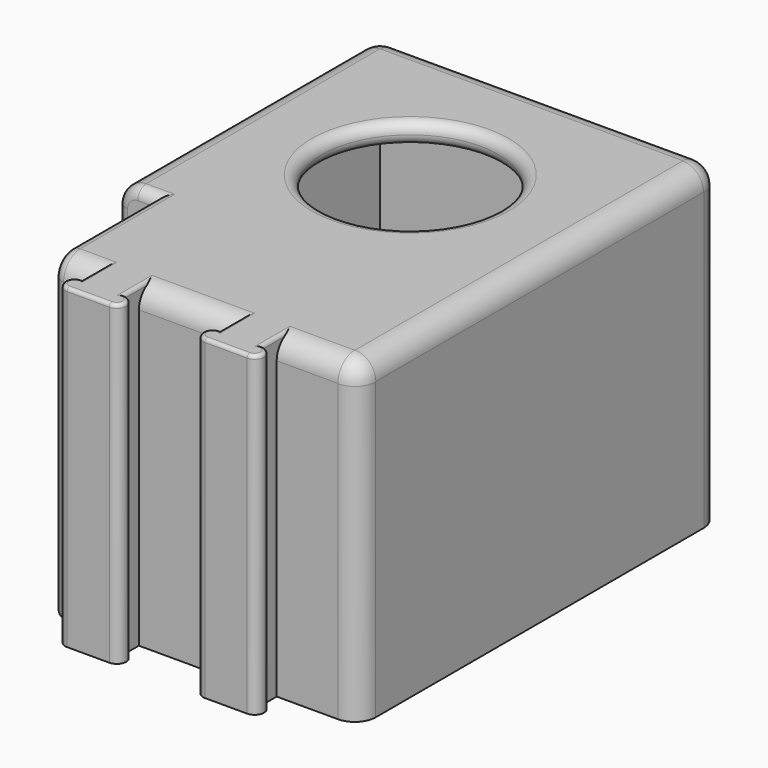
from build123d import *

# Parameters (mm, degrees)
F0_W           = 49
F0_H           = 49
F0_W_2         = 43
F0_H_2         = 43
F1_DEPTH       = 42
F2_DEPTH       = 3
F3_R           = 12.5
F4_DEPTH       = 3.001
F5_W           = 17
F5_H           = 13
F6_DEPTH       = 24.501
F8_DEPTH       = 42
F7_W           = 43
F7_H           = 12.25
F9_DEPTH       = 3
F11_DEPTH      = 3
F11_DEPTH_BACK = 42
F13_W          = 18.25
F13_H          = 45
F14_DEPTH      = 5.5
F15_T4_DEPTH   = 49.5024142802
F15_T9_DEPTH   = 48.0024142802
F15_T14_DEPTH  = 48.0024142802
F15_T19_DEPTH  = 49.5024142802
F15_T21_DEPTH  = 49.5014485948
F15_T23_DEPTH  = 50.5014485948
F15_T25_DEPTH  = 58.2480686292
F15_T27_DEPTH  = 42.9980686292
F15_T29_DEPTH  = 8.6990343146
F15_T31_DEPTH  = 13.7024142802
F15_T33_DEPTH  = 13.6
F15_S37_W      = 3.3015022539
F15_S37_H      = 3.3015022539
F15_T38_DEPTH  = 3.301502254
F15_S43_W      = 3.3015022539
F15_S43_H      = 3.3015022539
F15_T44_DEPTH  = 3.301502254
F15_S49_W      = 3.3015022539
F15_S49_H      = 3.3015022539
F15_T50_DEPTH  = 3.301502254
F15_T56_DEPTH  = 16.2014485948
F15_T61_DEPTH  = 21.2048285604
F15_T66_DEPTH  = 28.6048285604
F15_T71_DEPTH  = 28.6048285604
F16_R          = 1.49999
F17_R          = 1.5
F18_R          = 0.5


# Not quite as in the source:
# - a fillet or chamfer that OpenCascade refuses, or shapes differently, is made with other operations: its cross-section is extruded or revolved along the edge and cut away or added
# - a fillet or chamfer is up to 0.001 mm smaller than in the source, because OpenCascade refuses the exact size
# - a pattern or mirror of a feature is missing from the dataset's text; its kind, count and spacing are read off the source's solid


with BuildPart() as f1:
    # F0 (on Top) → F1 (new body)
    with BuildSketch(Plane.XY):
        Rectangle(F0_W, F0_H)
        Rectangle(F0_W_2, F0_H_2, mode=Mode.SUBTRACT)
    extrude(amount=-F1_DEPTH)

    # F0 (on Top) → F2 (join)
    with BuildSketch(Plane.XY):
        Rectangle(F0_W, F0_H)
        Rectangle(F0_W_2, F0_H_2, mode=Mode.SUBTRACT)
        Rectangle(F0_W_2, F0_H_2)
    extrude(amount=F2_DEPTH)

    # F3 (on Top) → F4 (cut, through all)
    with BuildSketch(Plane.XY):
        Circle(F3_R)
    extrude(amount=F4_DEPTH, mode=Mode.SUBTRACT)

    # F5 (on Front) → F6 (cut, through all)
    with BuildSketch(Plane.XZ):
        with Locations((0, -35.5)):
            Rectangle(F5_W, F5_H)
    extrude(amount=-F6_DEPTH, mode=Mode.SUBTRACT)

    # F7 (on Top) → F8 (join, through all)
    with BuildSketch(Plane.XY):
        Polygon((-21.5, -24.5), (-24.5, -24.5), (-24.5, -39.75), (24.5, -39.75), (24.5, -24.5), (21.5, -24.5), (21.5, -36.75), (-21.5, -36.75), align=None)
    extrude(amount=-F8_DEPTH)

    # F7 (on Top) → F9 (join, through all)
    with BuildSketch(Plane.XY):
        with Locations((0, -30.625)):
            Rectangle(F7_W, F7_H)
        Polygon((-21.5, -24.5), (-24.5, -24.5), (-24.5, -39.75), (24.5, -39.75), (24.5, -24.5), (21.5, -24.5), (21.5, -36.75), (-21.5, -36.75), align=None)
    extrude(amount=F9_DEPTH)

    # F10 (on Top) → F11 (join, two sides)
    with BuildSketch(Plane.XY) as f11_sk:
        with BuildLine():
            Line((12.8, -39.75), (6.8, -39.75))
            Line((6.8, -39.75), (6.8, -42.35))
            ThreePointArc((6.8, -42.35), (5.475, -43.675), (6.8, -45))
            Line((6.8, -45), (12.8, -45))
            ThreePointArc((12.8, -45), (14.125, -43.675), (12.8, -42.35))
            Line((12.8, -42.35), (12.8, -39.75))
        make_face()
    f11 = extrude(amount=F11_DEPTH) + extrude(f11_sk.sketch, amount=-F11_DEPTH_BACK)

    # F11_copies: F11 across plane
    add(f11.mirror(Plane(origin=(0, 0, 0), x_dir=(0, 0, -1), z_dir=(-1, 0, 0))))

    # F13 (on offset) → F14 (cut, through all)
    with BuildSketch(Plane.YZ.offset(-19)):
        with Locations((-30.625, -19.5)):
            Rectangle(F13_W, F13_H)
    extrude(amount=-F14_DEPTH, mode=Mode.SUBTRACT)

    # F15: fillet of radius 3 on 13 edges, made by hand


with BuildPart() as f15_tool2:
    # F15_s3 → F15_t4 (new body)
    with BuildSketch(Plane.XY.offset(7.5024142802)):
        with BuildLine():
            ThreePointArc((18.4990343146, -24.4996), (20.6213203436, -25.3786796564), (21.5004, -27.5009656854))
            Line((21.5004, -27.5009656854), (21.8005365685, -27.5009656854))
            ThreePointArc((21.8005365685, -27.5009656854), (21.8001365685, -26.0004828427), (21.8001365685, -24.5))
            Line((21.8001365685, -24.5), (21.5, -24.1998634315))
            ThreePointArc((21.5, -24.1998634315), (19.9995171573, -24.1998634315), (18.4990343146, -24.1994634315))
            Line((18.4990343146, -24.1994634315), (18.4990343146, -24.4996))
        make_face()
    extrude(amount=-F15_T4_DEPTH)

    split(bisect_by=Plane.XY.offset(3), keep=Keep.BOTTOM)


with BuildPart() as f1_1:
    add(f1.part)

    # F15_t1: union F15_tool2
    add(f15_tool2.part)


with BuildPart() as f15_tool7:
    # F15_s8 → F15_t9 (new body)
    with BuildSketch(Plane.YZ.offset(29.0024142802)):
        with BuildLine():
            ThreePointArc((-24.4996, -3.0009656854), (-25.3786796564, -0.8786796564), (-27.5009656854, 0.0004))
            Line((-27.5009656854, 0.0004), (-27.5009656854, 0.3005365685))
            ThreePointArc((-27.5009656854, 0.3005365685), (-26.0004828427, 0.3001365685), (-24.5, 0.3001365685))
            Line((-24.5, 0.3001365685), (-24.1998634315, 0))
            ThreePointArc((-24.1998634315, 0), (-24.1998634315, -1.5004828427), (-24.1994634315, -3.0009656854))
            Line((-24.1994634315, -3.0009656854), (-24.4996, -3.0009656854))
        make_face()
    extrude(amount=-F15_T9_DEPTH)

    split(bisect_by=Plane.YZ.offset(24.5), keep=Keep.BOTTOM)


with BuildPart() as f1_2:
    add(f1_1.part)

    # F15_t6: union F15_tool7
    add(f15_tool7.part)


with BuildPart() as f15_tool12:
    # F15_s13 → F15_t14 (new body)
    with BuildSketch(Plane.YZ.offset(29.0024142802)):
        with BuildLine():
            ThreePointArc((-33.7490343146, 0.0004), (-35.8713203436, -0.8786796564), (-36.7504, -3.0009656854))
            Line((-36.7504, -3.0009656854), (-37.0505365685, -3.0009656854))
            ThreePointArc((-37.0505365685, -3.0009656854), (-37.0501365685, -1.5004828427), (-37.0501365685, 0))
            Line((-37.0501365685, 0), (-36.75, 0.3001365685))
            ThreePointArc((-36.75, 0.3001365685), (-35.2495171573, 0.3001365685), (-33.7490343146, 0.3005365685))
            Line((-33.7490343146, 0.3005365685), (-33.7490343146, 0.0004))
        make_face()
    extrude(amount=-F15_T14_DEPTH)

    split(bisect_by=Plane.YZ.offset(24.5), keep=Keep.BOTTOM)


with BuildPart() as f1_3:
    add(f1_2.part)

    # F15_t11: union F15_tool12
    add(f15_tool12.part)


with BuildPart() as f15_tool17:
    # F15_s18 → F15_t19 (new body)
    with BuildSketch(Plane.XY.offset(7.5024142802)):
        with BuildLine():
            ThreePointArc((21.5004, -33.7490343146), (20.6213203436, -35.8713203436), (18.4990343146, -36.7504))
            Line((18.4990343146, -36.7504), (18.4990343146, -37.0505365685))
            ThreePointArc((18.4990343146, -37.0505365685), (19.9995171573, -37.0501365685), (21.5, -37.0501365685))
            Line((21.5, -37.0501365685), (21.8001365685, -36.75))
            ThreePointArc((21.8001365685, -36.75), (21.8001365685, -35.2495171573), (21.8005365685, -33.7490343146))
            Line((21.8005365685, -33.7490343146), (21.5004, -33.7490343146))
        make_face()
    extrude(amount=-F15_T19_DEPTH)

    split(bisect_by=Plane.XY.offset(3), keep=Keep.BOTTOM)


with BuildPart() as f1_4:
    add(f1_3.part)

    # F15_t16: union F15_tool17
    add(f15_tool17.part)

    # F15_s22 → F15_t21 (cut)
    with BuildSketch(Plane.XY.offset(-49.5024142802)):
        with BuildLine():
            ThreePointArc((21.4990343146, 24.5004), (23.6213203436, 23.6213203436), (24.5004, 21.4990343146))
            Line((24.5004, 21.4990343146), (24.8005365685, 21.4990343146))
            ThreePointArc((24.8005365685, 21.4990343146), (24.8001365685, 22.9995171573), (24.8001365685, 24.5))
            Line((24.8001365685, 24.5), (24.5, 24.8001365685))
            ThreePointArc((24.5, 24.8001365685), (22.9995171573, 24.8001365685), (21.4990343146, 24.8005365685))
            Line((21.4990343146, 24.8005365685), (21.4990343146, 24.5004))
        make_face()
        with BuildLine():
            ThreePointArc((-21.4990343146, 24.5004), (-23.6213203436, 23.6213203436), (-24.5004, 21.4990343146))
            Line((-24.5004, 21.4990343146), (-24.8005365685, 21.4990343146))
            ThreePointArc((-24.8005365685, 21.4990343146), (-24.8001365685, 22.9995171573), (-24.8001365685, 24.5))
            Line((-24.8001365685, 24.5), (-24.5, 24.8001365685))
            ThreePointArc((-24.5, 24.8001365685), (-22.9995171573, 24.8001365685), (-21.4990343146, 24.8005365685))
            Line((-21.4990343146, 24.8005365685), (-21.4990343146, 24.5004))
        make_face()
        with BuildLine():
            ThreePointArc((24.5004, -36.7490343146), (23.6213203436, -38.8713203436), (21.4990343146, -39.7504))
            Line((21.4990343146, -39.7504), (21.4990343146, -40.0505365685))
            ThreePointArc((21.4990343146, -40.0505365685), (22.9995171573, -40.0501365685), (24.5, -40.0501365685))
            Line((24.5, -40.0501365685), (24.8001365685, -39.75))
            ThreePointArc((24.8001365685, -39.75), (24.8001365685, -38.2495171573), (24.8005365685, -36.7490343146))
            Line((24.8005365685, -36.7490343146), (24.5004, -36.7490343146))
        make_face()
    extrude(amount=F15_T21_DEPTH, mode=Mode.SUBTRACT)

    # F15_s24 → F15_t23 (cut)
    with BuildSketch(Plane.XZ.offset(-21.4990343146)):
        with BuildLine():
            ThreePointArc((-21.4990343146, 3.0004), (-23.6213203436, 2.1213203436), (-24.5004, -0.0009656854))
            Line((-24.5004, -0.0009656854), (-24.8005365685, -0.0009656854))
            ThreePointArc((-24.8005365685, -0.0009656854), (-24.8001365685, 1.4995171573), (-24.8001365685, 3))
            Line((-24.8001365685, 3), (-24.5, 3.3001365685))
            ThreePointArc((-24.5, 3.3001365685), (-22.9995171573, 3.3001365685), (-21.4990343146, 3.3005365685))
            Line((-21.4990343146, 3.3005365685), (-21.4990343146, 3.0004))
        make_face()
    extrude(amount=F15_T23_DEPTH, mode=Mode.SUBTRACT)

    # F15_s26 → F15_t25 (cut)
    with BuildSketch(Plane.XZ.offset(-21.4990343146)):
        with BuildLine():
            ThreePointArc((24.5004, -0.0009656854), (23.6213203436, 2.1213203436), (21.4990343146, 3.0004))
            Line((21.4990343146, 3.0004), (21.4990343146, 3.3005365685))
            ThreePointArc((21.4990343146, 3.3005365685), (22.9995171573, 3.3001365685), (24.5, 3.3001365685))
            Line((24.5, 3.3001365685), (24.8001365685, 3))
            ThreePointArc((24.8001365685, 3), (24.8001365685, 1.4995171573), (24.8005365685, -0.0009656854))
            Line((24.8005365685, -0.0009656854), (24.5004, -0.0009656854))
        make_face()
    extrude(amount=F15_T25_DEPTH, mode=Mode.SUBTRACT)

    # F15_s28 → F15_t27 (cut)
    with BuildSketch(Plane.YZ.offset(-21.4990343146)):
        with BuildLine():
            ThreePointArc((24.5004, -0.0009656854), (23.6213203436, 2.1213203436), (21.4990343146, 3.0004))
            Line((21.4990343146, 3.0004), (21.4990343146, 3.3005365685))
            ThreePointArc((21.4990343146, 3.3005365685), (22.9995171573, 3.3001365685), (24.5, 3.3001365685))
            Line((24.5, 3.3001365685), (24.8001365685, 3))
            ThreePointArc((24.8001365685, 3), (24.8001365685, 1.4995171573), (24.8005365685, -0.0009656854))
            Line((24.8005365685, -0.0009656854), (24.5004, -0.0009656854))
        make_face()
    extrude(amount=F15_T27_DEPTH, mode=Mode.SUBTRACT)

    # F15_s30 → F15_t29 (cut)
    with BuildSketch(Plane.YZ.offset(12.8)):
        with BuildLine():
            ThreePointArc((-39.7504, -0.0009656854), (-38.8713203436, 2.1213203436), (-36.7490343146, 3.0004))
            Line((-36.7490343146, 3.0004), (-36.7490343146, 3.3005365685))
            ThreePointArc((-36.7490343146, 3.3005365685), (-38.2495171573, 3.3001365685), (-39.75, 3.3001365685))
            Line((-39.75, 3.3001365685), (-40.0501365685, 3))
            ThreePointArc((-40.0501365685, 3), (-40.0501365685, 1.4995171573), (-40.0505365685, -0.0009656854))
            Line((-40.0505365685, -0.0009656854), (-39.7504, -0.0009656854))
        make_face()
    extrude(amount=F15_T29_DEPTH, mode=Mode.SUBTRACT)

    # F15_s32 → F15_t31 (cut)
    with BuildSketch(Plane.YZ.offset(-26.5024142802)):
        with BuildLine():
            ThreePointArc((-39.7504, -0.0009656854), (-38.8713203436, 2.1213203436), (-36.7490343146, 3.0004))
            Line((-36.7490343146, 3.0004), (-36.7490343146, 3.3005365685))
            ThreePointArc((-36.7490343146, 3.3005365685), (-38.2495171573, 3.3001365685), (-39.75, 3.3001365685))
            Line((-39.75, 3.3001365685), (-40.0501365685, 3))
            ThreePointArc((-40.0501365685, 3), (-40.0501365685, 1.4995171573), (-40.0505365685, -0.0009656854))
            Line((-40.0505365685, -0.0009656854), (-39.7504, -0.0009656854))
        make_face()
    extrude(amount=F15_T31_DEPTH, mode=Mode.SUBTRACT)

    # F15_s34 → F15_t33 (cut)
    with BuildSketch(Plane.YZ.offset(-6.8)):
        with BuildLine():
            ThreePointArc((-39.7504, -0.0009656854), (-38.8713203436, 2.1213203436), (-36.7490343146, 3.0004))
            Line((-36.7490343146, 3.0004), (-36.7490343146, 3.3005365685))
            ThreePointArc((-36.7490343146, 3.3005365685), (-38.2495171573, 3.3001365685), (-39.75, 3.3001365685))
            Line((-39.75, 3.3001365685), (-40.0501365685, 3))
            ThreePointArc((-40.0501365685, 3), (-40.0501365685, 1.4995171573), (-40.0505365685, -0.0009656854))
            Line((-40.0505365685, -0.0009656854), (-39.7504, -0.0009656854))
        make_face()
    extrude(amount=F15_T33_DEPTH, mode=Mode.SUBTRACT)


with BuildPart() as f15_tool36:
    # F15_s37 → F15_t38 (new body)
    with BuildSketch(Plane.XY.offset(-0.0009656854)):
        with Locations((23.1497854416, 23.1497854416)):
            Rectangle(F15_S37_W, F15_S37_H)
    extrude(amount=F15_T38_DEPTH)

    # F15_s39 → F15_t40 (revolve, cut)
    with BuildSketch(Plane(origin=(21.4990343146, 21.4990343146, -0.0009656854), x_dir=(-0.7071067812, -0.7071067812, 0), z_dir=(-0.7071067812, 0.7071067812, 0))):
        with BuildLine():
            ThreePointArc((0, -3.0013656854), (3.0013656854, 0), (0, 3.0013656854))
            Line((0, 3.0013656854), (0, -3.0013656854))
        make_face()
    revolve(axis=Axis((21.4990343146, 21.4990343146, -0.0009656854), (0, 0, 1)), mode=Mode.SUBTRACT)


with BuildPart() as f1_5:
    add(f1_4.part)

    # F15_t35: cut F15_tool36
    add(f15_tool36.part, mode=Mode.SUBTRACT)


with BuildPart() as f15_tool42:
    # F15_s43 → F15_t44 (new body)
    with BuildSketch(Plane.XZ.offset(-21.4990343146)):
        with Locations((-23.1497854416, 1.6497854415)):
            Rectangle(F15_S43_W, F15_S43_H)
    extrude(amount=-F15_T44_DEPTH)

    # F15_s45 → F15_t46 (revolve, cut)
    with BuildSketch(Plane(origin=(-21.4990343146, 21.4990343146, -0.0009656854), x_dir=(0.7071067812, 0, -0.7071067812), z_dir=(0.7071067812, 0, 0.7071067812))):
        with BuildLine():
            ThreePointArc((0, -3.0013656854), (3.0013656854, 0), (0, 3.0013656854))
            Line((0, 3.0013656854), (0, -3.0013656854))
        make_face()
    revolve(axis=Axis((-21.4990343146, 21.4990343146, -0.0009656854), (0, 1, 0)), mode=Mode.SUBTRACT)


with BuildPart() as f1_6:
    add(f1_5.part)

    # F15_t41: cut F15_tool42
    add(f15_tool42.part, mode=Mode.SUBTRACT)


with BuildPart() as f15_tool48:
    # F15_s49 → F15_t50 (new body)
    with BuildSketch(Plane.XY.offset(-0.0009656854)):
        with Locations((23.1497854416, -38.3997854416)):
            Rectangle(F15_S49_W, F15_S49_H)
    extrude(amount=F15_T50_DEPTH)

    # F15_s51 → F15_t52 (revolve, cut)
    with BuildSketch(Plane(origin=(21.4990343146, -36.7490343146, -0.0009656854), x_dir=(-0.7071067812, 0.7071067812, 0), z_dir=(0.7071067812, 0.7071067812, 0))):
        with BuildLine():
            ThreePointArc((0, -3.0013656854), (3.0013656854, 0), (0, 3.0013656854))
            Line((0, 3.0013656854), (0, -3.0013656854))
        make_face()
    revolve(axis=Axis((21.4990343146, -36.7490343146, -0.0009656854), (0, 0, 1)), mode=Mode.SUBTRACT)


with BuildPart() as f1_7:
    add(f1_6.part)

    # F15_t47: cut F15_tool48
    add(f15_tool48.part, mode=Mode.SUBTRACT)


with BuildPart() as f15_tool54:
    # F15_s55 → F15_t56 (new body)
    with BuildSketch(Plane.YZ.offset(5.2975857198)):
        with BuildLine():
            ThreePointArc((-39.7504, -0.0009656854), (-38.8713203436, 2.1213203436), (-36.7490343146, 3.0004))
            Line((-36.7490343146, 3.0004), (-36.7490343146, 3.3005365685))
            ThreePointArc((-36.7490343146, 3.3005365685), (-38.2495171573, 3.3001365685), (-39.75, 3.3001365685))
            Line((-39.75, 3.3001365685), (-40.0501365685, 3))
            ThreePointArc((-40.0501365685, 3), (-40.0501365685, 1.4995171573), (-40.0505365685, -0.0009656854))
            Line((-40.0505365685, -0.0009656854), (-39.7504, -0.0009656854))
        make_face()
    extrude(amount=F15_T56_DEPTH)

    split(bisect_by=Plane.YZ.offset(6.8), keep=Keep.BOTTOM)


with BuildPart() as f1_8:
    add(f1_7.part)

    # F15_t53: cut F15_tool54
    add(f15_tool54.part, mode=Mode.SUBTRACT)


with BuildPart() as f15_tool59:
    # F15_s60 → F15_t61 (new body)
    with BuildSketch(Plane.YZ.offset(-26.5024142802)):
        with BuildLine():
            ThreePointArc((-39.7504, -0.0009656854), (-38.8713203436, 2.1213203436), (-36.7490343146, 3.0004))
            Line((-36.7490343146, 3.0004), (-36.7490343146, 3.3005365685))
            ThreePointArc((-36.7490343146, 3.3005365685), (-38.2495171573, 3.3001365685), (-39.75, 3.3001365685))
            Line((-39.75, 3.3001365685), (-40.0501365685, 3))
            ThreePointArc((-40.0501365685, 3), (-40.0501365685, 1.4995171573), (-40.0505365685, -0.0009656854))
            Line((-40.0505365685, -0.0009656854), (-39.7504, -0.0009656854))
        make_face()
    extrude(amount=F15_T61_DEPTH)

    split(bisect_by=Plane.YZ.offset(-6.8), keep=Keep.TOP)


with BuildPart() as f1_9:
    add(f1_8.part)

    # F15_t58: cut F15_tool59
    add(f15_tool59.part, mode=Mode.SUBTRACT)


with BuildPart() as f15_tool64:
    # F15_s65 → F15_t66 (new body)
    with BuildSketch(Plane.YZ.offset(-14.3024142802)):
        with BuildLine():
            ThreePointArc((-39.7504, -0.0009656854), (-38.8713203436, 2.1213203436), (-36.7490343146, 3.0004))
            Line((-36.7490343146, 3.0004), (-36.7490343146, 3.3005365685))
            ThreePointArc((-36.7490343146, 3.3005365685), (-38.2495171573, 3.3001365685), (-39.75, 3.3001365685))
            Line((-39.75, 3.3001365685), (-40.0501365685, 3))
            ThreePointArc((-40.0501365685, 3), (-40.0501365685, 1.4995171573), (-40.0505365685, -0.0009656854))
            Line((-40.0505365685, -0.0009656854), (-39.7504, -0.0009656854))
        make_face()
    extrude(amount=F15_T66_DEPTH)

    split(bisect_by=Plane.YZ.offset(-12.8), keep=Keep.BOTTOM)


with BuildPart() as f1_10:
    add(f1_9.part)

    # F15_t63: cut F15_tool64
    add(f15_tool64.part, mode=Mode.SUBTRACT)


with BuildPart() as f15_tool69:
    # F15_s70 → F15_t71 (new body)
    with BuildSketch(Plane.YZ.offset(-14.3024142802)):
        with BuildLine():
            ThreePointArc((-39.7504, -0.0009656854), (-38.8713203436, 2.1213203436), (-36.7490343146, 3.0004))
            Line((-36.7490343146, 3.0004), (-36.7490343146, 3.3005365685))
            ThreePointArc((-36.7490343146, 3.3005365685), (-38.2495171573, 3.3001365685), (-39.75, 3.3001365685))
            Line((-39.75, 3.3001365685), (-40.0501365685, 3))
            ThreePointArc((-40.0501365685, 3), (-40.0501365685, 1.4995171573), (-40.0505365685, -0.0009656854))
            Line((-40.0505365685, -0.0009656854), (-39.7504, -0.0009656854))
        make_face()
    extrude(amount=F15_T71_DEPTH)

    split(bisect_by=Plane.YZ.offset(12.8), keep=Keep.TOP)


with BuildPart() as f1_11:
    add(f1_10.part)

    # F15_t68: cut F15_tool69
    add(f15_tool69.part, mode=Mode.SUBTRACT)

    # F16 (radius 1.5 in the source; OpenCascade refuses exactly that, so slightly less here)
    f16_edges = [f1_11.edges().sort_by_distance(p)[0] for p in [
        (-12.5, 0, 0),
        (12.5, 0, 1.5),
        (-12.5, 0, 3),
    ]]
    fillet(f16_edges, radius=F16_R)

    # F17
    f17_edges = [f1_11.edges().sort_by_distance(p)[0] for p in [
        (-19, -38.25, -42),
        (-19, -29.149017, 3),
        (-20.274017, -21.5, 3),
        (-23, -21.5, -42),
        (-19, -23, -42),
        (-23.62132, -21.5, 2.12132),
        (-24.5, -21.5, -20.975983),
        (-19, -39.75, -20.975983),
        (-19, -38.87132, 2.12132),
        (-8.5, 23, -42),
        (8.5, 23, -42),
        (-8.5, 23, -29),
        (8.5, 23, -29),
    ]]
    fillet(f17_edges, radius=F17_R)

    # F18
    f18_edges = [f1_11.edges().sort_by_distance(p)[0] for p in [
        (5.475, -43.675, 3),
        (6.8, -39.574017, 3),
        (12.8, -39.574017, 3),
        (14.125, -43.675, 3),
        (9.8, -45, 3),
        (-12.8, -39.574017, 3),
        (-14.125, -43.675, 3),
        (-9.8, -45, 3),
        (-5.475, -43.675, 3),
        (-6.8, -39.574017, 3),
    ]]
    fillet(f18_edges, radius=F18_R)


solid = f1_11.part
